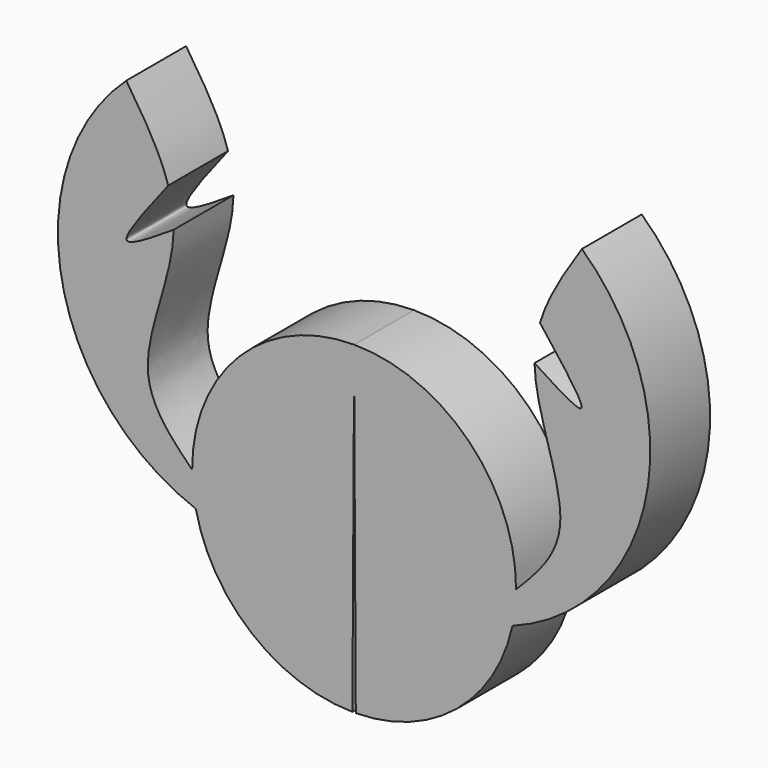
from build123d import *

# Parameters (mm, degrees)
F1_DEPTH = 12.7


with BuildPart() as f1:
    # F0 (on Front) → F1 (new body)
    with BuildSketch(Plane.XZ):
        with BuildLine():
            add(Edge.make_bspline(
                [(-38.6931858957, 54.3991737068), (-35.8405403413, 50.0610999657), (-32.9878947868, 45.7230262247), (-31.5682335133, 41.0291340153)],
                knots=[0, 0, 0, 0, 0.2439114114, 0.2439114114, 0.2439114114, 0.2439114114], degree=3))
            ThreePointArc((-38.6931858957, 54.3991737068), (-49.6350522053, 21.0007464247), (-26.8898194638, -5.7916736001))
            ThreePointArc((-26.8898194638, -5.7916736001), (-17.3939863098, -21.3085690308), (-0.2898975187, -27.5049419798))
            Line((-0.2898975187, -27.5049419798), (0.0159435843, 27.5064650525))
            ThreePointArc((0.0159435843, 27.5064650525), (-19.4983805085, 19.401521369), (-27.5060445831, -0.1529224477))
            add(Edge.make_bspline(
                [(-30.6462217122, 34.7148962319), (-30.7754650722, 27.1593597), (-39.1689548904, 11.6131795075), (-31.0760950053, 3.448715235), (-27.5060445831, -0.1529224477)],
                knots=[0.3493301375, 0.3493301375, 0.3493301375, 0.3493301375, 0.7129662134, 1, 1, 1, 1], degree=3))
            add(Edge.make_bspline(
                [(-31.5682335133, 41.0291340153), (-35.3674367785, 36.1399617518), (-42.4430865557, 27.1135638958), (-34.3396168251, 32.3313583593), (-30.6462217122, 34.7148962319)],
                knots=[0, 0, 0, 0, 0.5426319314, 1, 1, 1, 1], degree=3))
        make_face()
    extrude(amount=F1_DEPTH)

    # F2: F1 across plane


with BuildPart() as f1_1:
    add(f1.part)
    add(f1.part.mirror(Plane.YZ))


solid = f1_1.part
